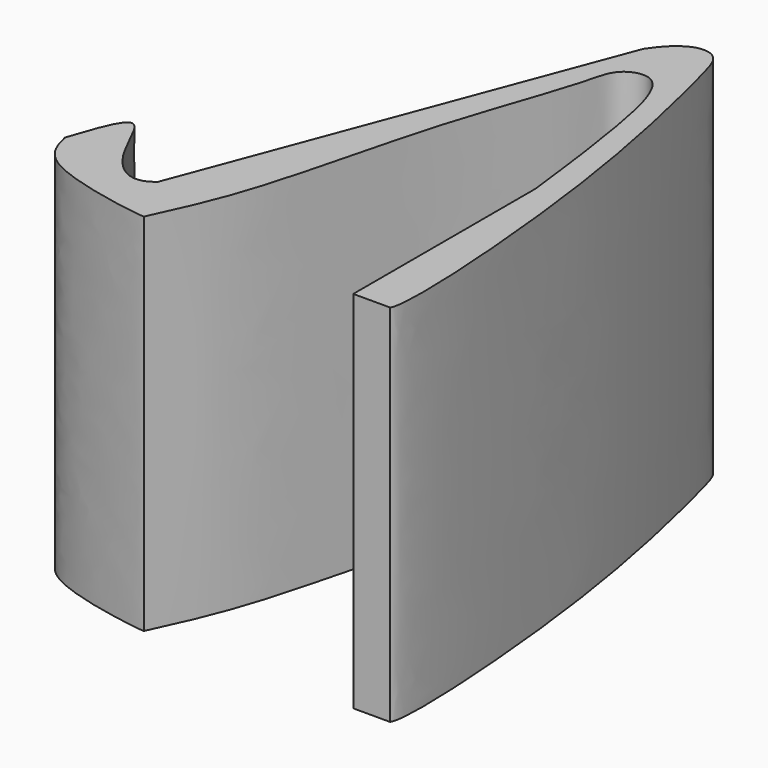
from build123d import *

# Parameters (mm, degrees)
F1_DEPTH = 50


with BuildPart() as f1:
    # F0 (on Top) → F1 (new body)
    with BuildSketch(Plane.XY):
        with BuildLine():
            add(Edge.make_bspline(
                [(0, 9.0214600787), (1.1979784843, 12.6373479056), (3.5960097678, 19.8753845147), (6.8442783914, 8.4855962552), (11.8172982842, 5.1384805823), (14.1977071762, 7.2467466816)],
                knots=[0, 0, 0, 0, 0.0854832851, 0.1711145855, 0.250406668, 0.250406668, 0.250406668, 0.250406668], degree=3))
            add(Edge.make_bspline(
                [(0, 9.0214600787), (0.4707372138, 7.1082883365), (1.6542648588, 2.2981913651), (17.6040614268, -0.0730355148), (17.9943904396, -0.0080766626), (18.04292202, 0)],
                knots=[0, 0, 0, 0, 0.3664076644, 0.9212222603, 1, 1, 1, 1], degree=3))
            add(Edge.make_bspline(
                [(18.04292202, 0), (19.7640667697, 3.6785597698), (23.8398330825, 12.3895935112), (28.8054917195, 35.8260900341), (35.3620501424, 52.9226470966), (36.1277778893, 58.4277478561), (41.9881309739, 60.1625625139), (44.8259980884, 47.1846563473), (46.052296735, 36.9152090584), (46.7341206968, 31.2053803355)],
                knots=[0, 0, 0, 0, 0.148815075, 0.3524023587, 0.5273547018, 0.6166730489, 0.6941809116, 0.8299641095, 1, 1, 1, 1], degree=3))
            add(Edge.make_bspline(
                [(46.7341206968, 31.2053803355), (46.7341206968, 20.8035868903), (46.7341206968, 10.4017934452), (46.7341206968, 0)],
                knots=[0, 0, 0, 0, 31.2053803355, 31.2053803355, 31.2053803355, 31.2053803355], degree=3))
            Line((46.7341206968, 0), (51.1709041893, 0))
            Line((51.1709041893, 0), (51.7624765635, 0))
            add(Edge.make_bspline(
                [(35.4942716658, 63.7417957187), (38.0288123619, 67.6273778401), (42.6210871493, 68.4190440537), (44.4981634124, 61.782518195), (50.8994915627, 36.0690092341), (53.0389515253, 1.4447194238), (51.7624765635, 0)],
                knots=[0.4861779531, 0.4861779531, 0.4861779531, 0.4861779531, 0.5687889606, 0.6340779311, 0.8007283318, 0.9766620077, 0.9766620077, 0.9766620077, 0.9766620077], degree=3))
            Line((35.4942716658, 63.7417957187), (27.0593505178, 41.3658259179))
            add(Edge.make_bspline(
                [(14.1977071762, 7.2467466816), (18.4937417846, 11.0516325384), (22.7554914057, 26.9648141089), (27.0593505178, 41.3658259179)],
                knots=[0.250406668, 0.250406668, 0.250406668, 0.250406668, 0.3935087762, 0.3935087762, 0.3935087762, 0.3935087762], degree=3))
        make_face()
        with BuildLine():
            Line((27.0593505178, 41.3658259179), (14.1977071762, 7.2467466816))
            add(Edge.make_bspline(
                [(14.1977071762, 7.2467466816), (18.4937417846, 11.0516325384), (22.7554914057, 26.9648141089), (27.0593505178, 41.3658259179)],
                knots=[0.250406668, 0.250406668, 0.250406668, 0.250406668, 0.3935087762, 0.3935087762, 0.3935087762, 0.3935087762], degree=3))
        make_face()
    extrude(amount=F1_DEPTH)


solid = f1.part
